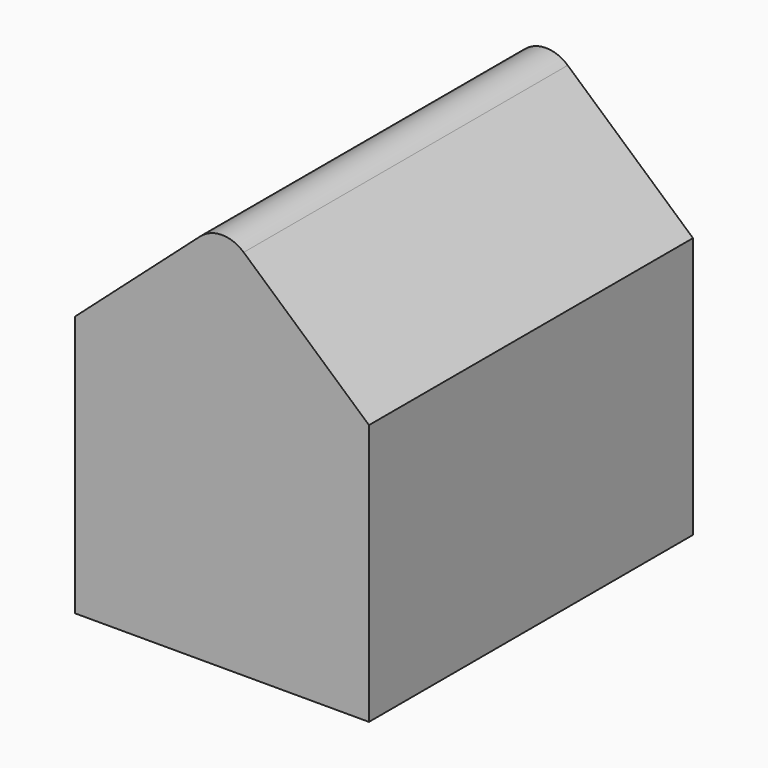
from build123d import *

# Parameters (mm, degrees)
F0_W     = 9
F0_H     = 12.4
F1_DEPTH = 4
F2_W     = 9
F2_H     = 12.4
F3_DEPTH = 4
F5_DEPTH = 12.4
F6_R     = 1


with BuildPart() as f1:
    # F0 (on Top) → F1 (new body)
    with BuildSketch(Plane.XY):
        with Locations((-4.5, -6.2)):
            Rectangle(F0_W, F0_H)
    extrude(amount=F1_DEPTH)

    # F2 (on face) → F3 (join)
    with BuildSketch(Plane.XY.offset(4)):
        with Locations((-4.5, -6.2)):
            Rectangle(F2_W, F2_H)
    extrude(amount=F3_DEPTH)

    # F4 (on face) → F5 (join, through all)
    with BuildSketch(Plane.XZ.offset(12.4)):
        Polygon((-4.5, 12), (-9, 8), (0, 8), align=None)
    extrude(amount=-F5_DEPTH)

    # F6
    f6_edges = [f1.edges().sort_by_distance(p)[0] for p in [
        (-4.5, -6.2, 12),
    ]]
    fillet(f6_edges, radius=F6_R)


solid = f1.part
